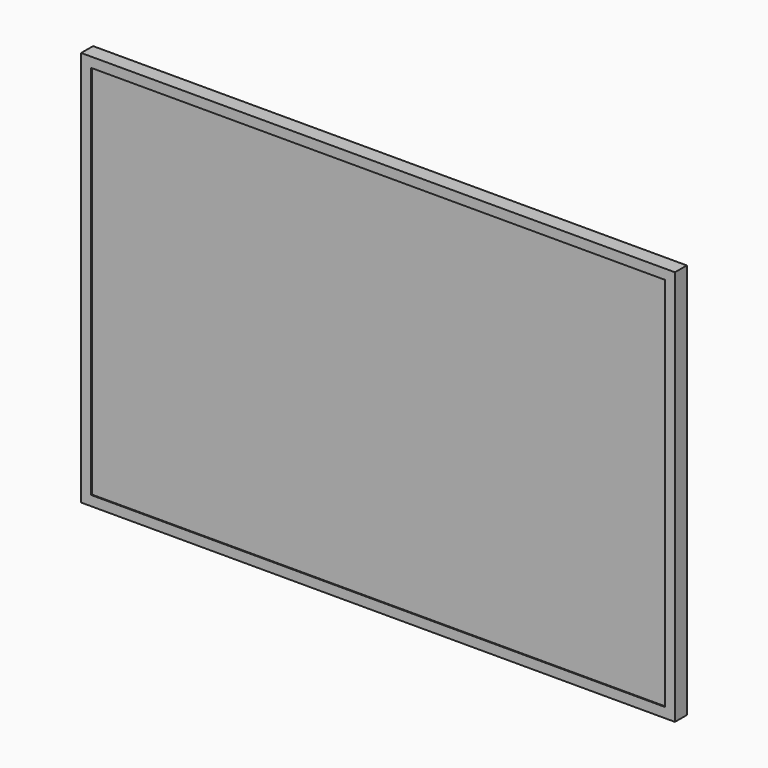
from build123d import *

# Parameters (mm, degrees)
F0_W         = 600
F0_H         = 400
F0_W_2       = 580
F0_H_2       = 380
F1_DEPTH     = 15
F2_W         = 580
F2_H         = 380
F3_DEPTH     = 1
F4_R         = 35
F5_DEPTH     = 7
F6_TEXT_SIZE = 47.2760849492
F7_DEPTH     = 5


# Not quite as in the source:
# - Text() gives the source's letters only with a copy of the font that has no kerning and outlines rounded to 1/6400 em; it was checked with that copy


with BuildPart() as f1:
    # F0 (on Front) → F1 (new body)
    with BuildSketch(Plane.XZ):
        with Locations((0, 200)):
            Rectangle(F0_W, F0_H)
        with Locations((0, 200)):
            Rectangle(F0_W_2, F0_H_2, mode=Mode.SUBTRACT)
        with Locations((0, 200)):
            Rectangle(F0_W_2, F0_H_2)
    extrude(amount=F1_DEPTH)

    # F2 (on face) → F3 (cut)
    with BuildSketch(Plane.XZ.offset(15)):
        with Locations((0, 200)):
            Rectangle(F2_W, F2_H)
    extrude(amount=-F3_DEPTH, mode=Mode.SUBTRACT)

    # F4 (on face) → F5 (cut)
    with BuildSketch(Plane(origin=(0, 0, 0), x_dir=(-1, 0, 0), z_dir=(0, 1, 0))):
        with Locations((0, 150)):
            Circle(F4_R)
    extrude(amount=-F5_DEPTH, mode=Mode.SUBTRACT)

    # F6 (on face) → F7 (join)
    with BuildSketch(Plane(origin=(0, 0, 0), x_dir=(-1, 0, 0), z_dir=(0, 1, 0))):
        with Locations((-100, 265.9612188366)):
            Text('Jang yo a', F6_TEXT_SIZE, font='Open Sans', text_align=(TextAlign.LEFT, TextAlign.BOTTOM))
    extrude(amount=F7_DEPTH)


solid = f1.part
